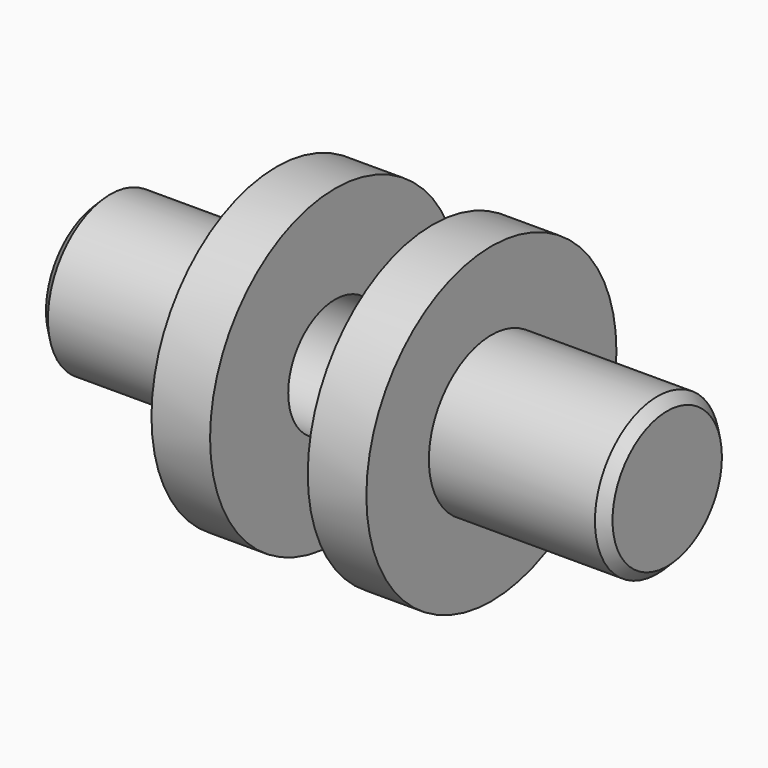
from build123d import *

# Parameters (mm, degrees)
F0_R     = 203.2
F1_DEPTH = 609.6
F3_D     = 304.8
F3_DEPTH = 508
F3_TIP   = 91.5711583398
F0_R_2   = 406.4
F4_DEPTH = 152.4
F5_SIZE2 = 25.4
F5_SIZE  = 25.4


# Not quite as in the source:
# - a feature names something its author has since deleted; it is built from what else it names


with BuildPart() as f1:
    # F0 (on Right) → F1 (new body)
    with BuildSketch(Plane.YZ):
        Circle(F0_R)
    extrude(amount=-F1_DEPTH)

    # F3
    with Locations(Plane.YZ):
        with Locations((0, 0)):
            Hole(F3_D / 2, depth=F3_DEPTH)
            with Locations((0, 0, -(F3_DEPTH + F3_TIP / 2))):  # 118° drill point
                Cone(0, F3_D / 2, F3_TIP, mode=Mode.SUBTRACT)

    # F0 (on Right) → F4 (join)
    with BuildSketch(Plane.YZ):
        Circle(F0_R_2)
        Circle(F0_R, mode=Mode.SUBTRACT)
    extrude(amount=-F4_DEPTH)

    # F5
    f5_edges = [f1.edges().sort_by_distance(p)[0] for p in [
        (-609.6, -203.2, 0),
    ]]
    chamfer(f5_edges, length=F5_SIZE, length2=F5_SIZE2)


with BuildPart() as f7_1:
    # F7: instance of F1
    add(f1.part.mirror(Plane.YZ.offset(127)))


solid = Compound([f1.part, f7_1.part])
